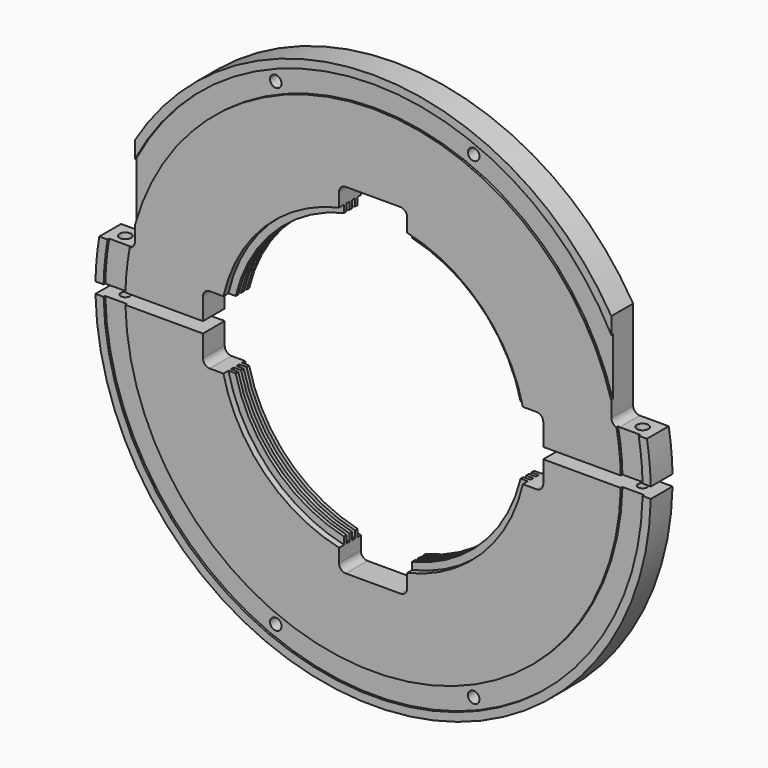
from build123d import *

# Parameters (mm, degrees)
F2_W     = 79
F2_H     = 8
F2_W_2   = 100
F2_H_2   = 21
F2_W_3   = 50
F2_H_3   = 100
F2_W_4   = 80
F2_H_4   = 80
F2_R     = 4.25
F3_DEPTH = 25
F5_D     = 6.8
F5_DEPTH = 22
F5_START = 4
F5_TIP   = 2.0429261047
F6_D     = 8.5
F6_DEPTH = 204.001
F7_R     = 5


with BuildPart() as f1:
    # F0 (on Right) → F1 (revolve)
    with BuildSketch(Plane.YZ):
        Polygon((20, 204), (0, 204), (0, 198), (1.5, 198), (1.5, 182), (0, 182), (0, 112.8), (4.6, 112.8), (4.6, 107.6), (7, 107.6), (7, 112.8), (9.6, 112.8), (9.6, 107.6), (12, 107.6), (12, 112.8), (14.6, 112.8), (14.6, 107.6), (17, 107.6), (17, 112.8), (20, 112.8), align=None)
    revolve(axis=Axis((0, 10, 0), (0, 1, 0)))

    # F2 (on Front) → F3 (cut)
    with BuildSketch(Plane.XZ):
        with Locations((-164.5, 0)):
            Rectangle(F2_W, F2_H)
        with Locations((-75, 14.5)):
            Rectangle(F2_W_2, F2_H_2)
        with Locations((-75, 0)):
            Rectangle(F2_W_2, F2_H)
        with Locations((0, 14.5)):
            Rectangle(F2_W_3, F2_H_2)
        with Locations((-75, -14.5)):
            Rectangle(F2_W_2, F2_H_2)
        with Locations((75, 14.5)):
            Rectangle(F2_W_2, F2_H_2)
        with Locations((75, 0)):
            Rectangle(F2_W_2, F2_H)
        with Locations((0, 75)):
            Rectangle(F2_W_3, F2_H_3)
        with Locations((0, -14.5)):
            Rectangle(F2_W_3, F2_H_2)
        with Locations((164.5, 0)):
            Rectangle(F2_W, F2_H)
        with Locations((75, -14.5)):
            Rectangle(F2_W_2, F2_H_2)
        with Locations((0, -75)):
            Rectangle(F2_W_3, F2_H_3)
        with Locations((-215, 74)):
            Rectangle(F2_W_4, F2_H_4)
        with Locations((215, 74)):
            Rectangle(F2_W_4, F2_H_4)
        with Locations((-72.7098521494, 175.5371111771)):
            Circle(F2_R)
        with Locations((72.7098521494, 175.5371111771)):
            Circle(F2_R)
        with Locations((-72.7098521494, -175.5371111771)):
            Circle(F2_R)
        with Locations((72.7098521494, -175.5371111771)):
            Circle(F2_R)
    extrude(amount=-F3_DEPTH, mode=Mode.SUBTRACT)

    # F5
    # its depths count from where the whole tool has entered the part; down to there all is cleared
    with Locations(Plane.XY.offset(-F5_START)):
        with Locations((-190, 10), (190, 10)):
            Hole(F5_D / 2, depth=F5_DEPTH)
            with Locations((0, 0, -(F5_DEPTH + F5_TIP / 2))):  # 118° drill point
                Cone(0, F5_D / 2, F5_TIP, mode=Mode.SUBTRACT)

    # F6 (through all, one way)
    with BuildSketch(Plane(origin=(0, 0, 0), x_dir=(1, 0, 0), z_dir=(0, 0, -1))):
        with Locations((-190, -10), (190, -10)):
            Circle(F6_D / 2)
    extrude(amount=-F6_DEPTH, mode=Mode.SUBTRACT)

    # F7
    f7_edges = [f1.edges().sort_by_distance(p)[0] for p in [
        (-125, 10, -25),
        (-125, 10, 25),
        (-25, 10, 125),
        (25, 10, 125),
        (125, 10, 25),
        (125, 10, -25),
        (25, 10, -125),
        (-25, 10, -125),
        (-175, 10, 34),
        (175, 10, 34),
    ]]
    fillet(f7_edges, radius=F7_R)


solid = f1.part
